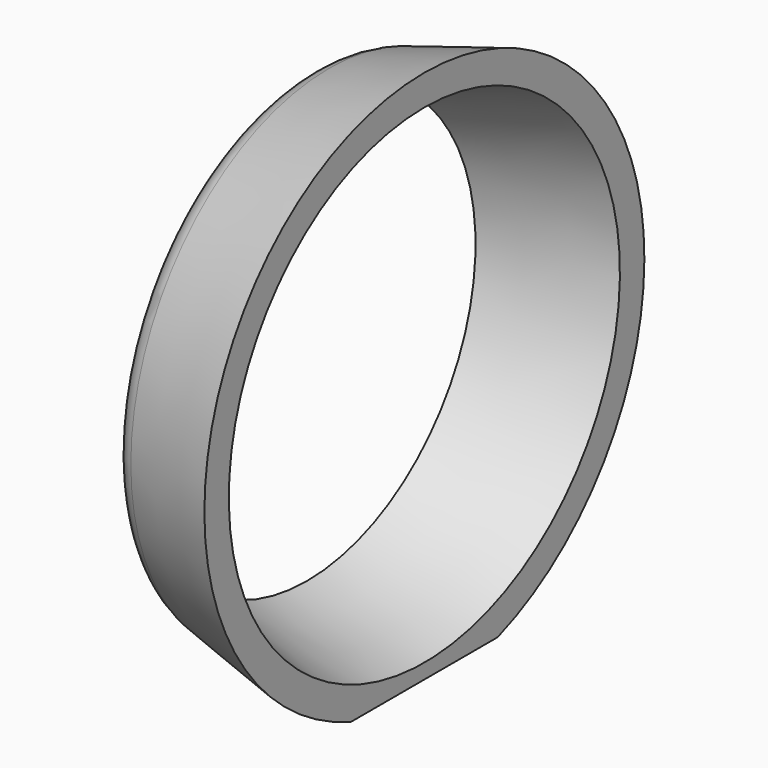
from build123d import *

# Parameters (mm, degrees)
F2_W     = 50
F2_H     = 12.9609592259
F3_DEPTH = 35.1
F4_R     = 5


# Not quite as in the source:
# - a feature names something its author has since deleted; it is built from what else it names


with BuildPart() as f1:
    # F0 (on Front) → F1 (revolve)
    with BuildSketch(Plane.XZ):
        Polygon((-52.483901754, 46.9848437961), (-52.483901754, 41.9848437961), (-33.255017231, 47.4848437961), (-33.255017231, 52.4848437961), align=None)
    revolve(axis=Axis((-42.8694594925, 0, 7.4848437961), (1, 0, 0)))

    # F2 (on Front) → F3 (cut, symmetric)
    with BuildSketch(Plane.XZ):
        with Locations((-24.5732873678, -41.422042688)):
            Rectangle(F2_W, F2_H)
    extrude(amount=F3_DEPTH, both=True, mode=Mode.SUBTRACT)

    # F4
    f4_edges = [f1.edges().sort_by_distance(p)[0] for p in [
        (-52.483902, 0, -32.015156),
    ]]
    fillet(f4_edges, radius=F4_R)


solid = f1.part
